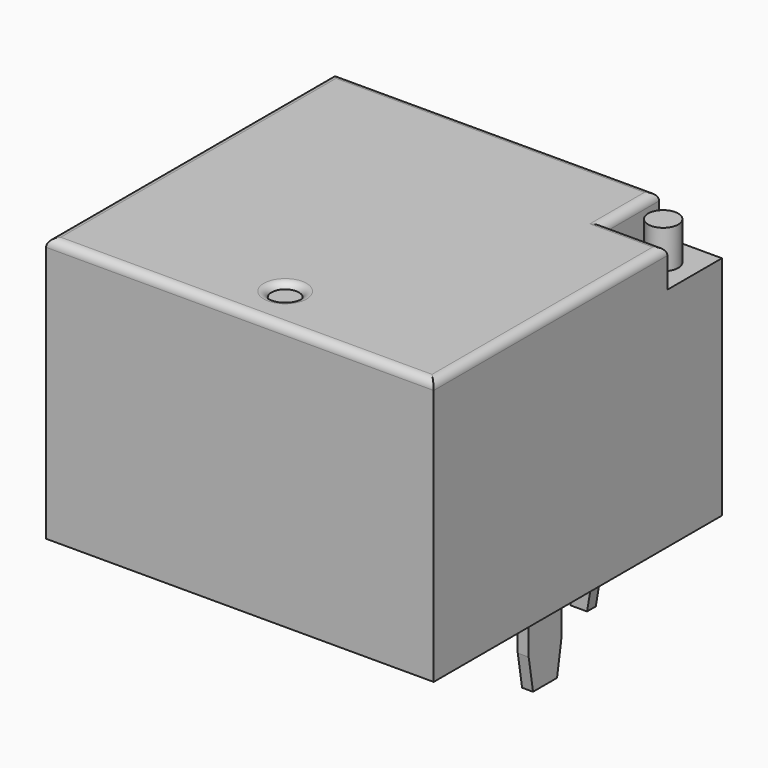
from build123d import *

# Parameters (mm, degrees)
F1_W         = 14.2
F1_H         = 13.2
F2_DEPTH     = 9.7
F0_W         = 0.4
F0_H         = 1.5
F3_DEPTH     = 3.5
F0_W_2       = 1.5
F0_H_2       = 0.4
F0_W_3       = 1
F4_W         = 2.3
F4_H         = 2.5
F4_R         = 0.55
F5_DEPTH     = 1.4
F4_R_2       = 0.5
F6_DEPTH     = 0.2
F7_T1_DEPTH  = 3.25
F7_T3_DEPTH  = 13.4
F7_T5_DEPTH  = 3.05
F7_T7_DEPTH  = 14.7
F7_T9_DEPTH  = 12.2
F7_T11_DEPTH = 15.7
F7_T19_DEPTH = 3.25
F7_T23_DEPTH = 3.05
F8_SIZE2     = 1.2
F8_SIZE      = 0.2
F8_2_SIZE2   = 1.2
F8_2_SIZE    = 0.2
F8_3_SIZE2   = 1.2
F8_3_SIZE    = 0.2
F8_4_SIZE2   = 1.2
F8_4_SIZE    = 0.2
F8_5_SIZE2   = 1.2
F8_5_SIZE    = 0.2


# Not quite as in the source:
# - a fillet or chamfer that OpenCascade refuses, or shapes differently, is made with other operations: its cross-section is extruded or revolved along the edge and cut away or added


with BuildPart() as f2:
    # F1 (on Top) → F2 (new body)
    with BuildSketch(Plane.XY):
        with Locations((-0.3, -0.5)):
            Rectangle(F1_W, F1_H)
    extrude(amount=F2_DEPTH)

    # F4 (on face) → F5 (cut)
    with BuildSketch(Plane.XY.offset(9.7)):
        with Locations((5.65, 4.85)):
            Rectangle(F4_W, F4_H)
        with Locations((5.65, 4.85)):
            Circle(F4_R, mode=Mode.SUBTRACT)
    extrude(amount=-F5_DEPTH, mode=Mode.SUBTRACT)

    # F4 (on face) → F6 (cut)
    with BuildSketch(Plane.XY.offset(9.7)):
        with Locations((0, -5.4)):
            Circle(F4_R_2)
    extrude(amount=-F6_DEPTH, mode=Mode.SUBTRACT)

    # F7: fillet of radius 0.3 on 7 edges, made by hand

    # F7_s2 → F7_t1 (cut)
    with BuildSketch(Plane.XZ.offset(-6.85)):
        with BuildLine():
            ThreePointArc((4.2, 9.7), (4.4121320344, 9.6121320344), (4.5, 9.4))
            Line((4.5, 9.4), (4.5, 9.7))
            Line((4.5, 9.7), (4.2, 9.7))
        make_face()
    extrude(amount=F7_T1_DEPTH, mode=Mode.SUBTRACT)

    # F7_s4 → F7_t3 (cut)
    with BuildSketch(Plane.YZ.offset(-8.15)):
        with BuildLine():
            ThreePointArc((6.1, 9.4), (6.0121320344, 9.6121320344), (5.8, 9.7))
            Line((5.8, 9.7), (6.1, 9.7))
            Line((6.1, 9.7), (6.1, 9.4))
        make_face()
    extrude(amount=F7_T3_DEPTH, mode=Mode.SUBTRACT)

    # F7_s6 → F7_t5 (cut)
    with BuildSketch(Plane.YZ.offset(4.5)):
        with BuildLine():
            ThreePointArc((3.3, 9.7), (3.5121320344, 9.6121320344), (3.6, 9.4))
            Line((3.6, 9.4), (3.6, 9.7))
            Line((3.6, 9.7), (3.3, 9.7))
        make_face()
    extrude(amount=F7_T5_DEPTH, mode=Mode.SUBTRACT)

    # F7_s8 → F7_t7 (cut)
    with BuildSketch(Plane.XZ.offset(-6.85)):
        with BuildLine():
            ThreePointArc((-7.4, 9.4), (-7.3121320344, 9.6121320344), (-7.1, 9.7))
            Line((-7.1, 9.7), (-7.4, 9.7))
            Line((-7.4, 9.7), (-7.4, 9.4))
        make_face()
    extrude(amount=F7_T7_DEPTH, mode=Mode.SUBTRACT)

    # F7_s10 → F7_t9 (cut)
    with BuildSketch(Plane.XZ.offset(-4.35)):
        with BuildLine():
            ThreePointArc((6.5, 9.7), (6.7121320344, 9.6121320344), (6.8, 9.4))
            Line((6.8, 9.4), (6.8, 9.7))
            Line((6.8, 9.7), (6.5, 9.7))
        make_face()
    extrude(amount=F7_T9_DEPTH, mode=Mode.SUBTRACT)

    # F7_s12 → F7_t11 (cut)
    with BuildSketch(Plane.YZ.offset(-8.15)):
        with BuildLine():
            ThreePointArc((-6.8, 9.7), (-7.0121320344, 9.6121320344), (-7.1, 9.4))
            Line((-7.1, 9.4), (-7.1, 9.7))
            Line((-7.1, 9.7), (-6.8, 9.7))
        make_face()
    extrude(amount=F7_T11_DEPTH, mode=Mode.SUBTRACT)

    # F7_s13 → F7_t14 (revolve, cut)
    with BuildSketch(Plane.XZ.offset(5.4)):
        with BuildLine():
            ThreePointArc((0.7828427125, 9.7), (0.6096376317, 9.6449489743), (0.5, 9.5))
            Line((0.5, 9.5), (0.5, 9.7))
            Line((0.5, 9.7), (0.7828427125, 9.7))
        make_face()
    revolve(axis=Axis((0, -5.4, 9.7), (0, 0, 1)), mode=Mode.SUBTRACT)


with BuildPart() as f3:
    # F0 (on Top) → F3 (new body)
    with BuildSketch(Plane.XY):
        with Locations((-5.7, 0)):
            Rectangle(F0_W, F0_H)
    extrude(amount=-F3_DEPTH)

    # F8
    f8_edges = [f3.edges().sort_by_distance(p)[0] for p in [
        (-5.7, -0.75, -3.5),
        (-5.7, 0.75, -3.5),
    ]]
    f8_side = f3.faces().sort_by_distance((-5.7, 0, -3.5))[0]
    chamfer(f8_edges, length=F8_SIZE, length2=F8_SIZE2, reference=f8_side)


with BuildPart() as f3b:
    # F0 (on Top) → F3, piece 2 (new body)
    with BuildSketch(Plane.XY):
        with Locations((5, 0)):
            Rectangle(F0_W, F0_H)
    extrude(amount=-F3_DEPTH)

    # F8#5
    f8_5_edges = [f3b.edges().sort_by_distance(p)[0] for p in [
        (5, -0.75, -3.5),
        (5, 0.75, -3.5),
    ]]
    f8_5_side = f3b.faces().sort_by_distance((5, 0, -3.5))[0]
    chamfer(f8_5_edges, length=F8_5_SIZE, length2=F8_5_SIZE2, reference=f8_5_side)


with BuildPart() as f3c:
    # F0 (on Top) → F3, piece 3 (new body)
    with BuildSketch(Plane.XY):
        with Locations((0, -5.4)):
            Rectangle(F0_W_2, F0_H_2)
    extrude(amount=-F3_DEPTH)

    # F8#2
    f8_2_edges = [f3c.edges().sort_by_distance(p)[0] for p in [
        (0.75, -5.4, -3.5),
        (-0.75, -5.4, -3.5),
    ]]
    f8_2_side = f3c.faces().sort_by_distance((0, -5.4, -3.5))[0]
    chamfer(f8_2_edges, length=F8_2_SIZE, length2=F8_2_SIZE2, reference=f8_2_side)


with BuildPart() as f3d:
    # F0 (on Top) → F3, piece 4 (new body)
    with BuildSketch(Plane.XY):
        with Locations((-3, 4.5)):
            Rectangle(F0_W_3, F0_H_2)
    extrude(amount=-F3_DEPTH)

    # F8#3
    f8_3_edges = [f3d.edges().sort_by_distance(p)[0] for p in [
        (-2.5, 4.5, -3.5),
        (-3.5, 4.5, -3.5),
    ]]
    f8_3_side = f3d.faces().sort_by_distance((-3, 4.5, -3.5))[0]
    chamfer(f8_3_edges, length=F8_3_SIZE, length2=F8_3_SIZE2, reference=f8_3_side)


with BuildPart() as f3e:
    # F0 (on Top) → F3, piece 5 (new body)
    with BuildSketch(Plane.XY):
        with Locations((3, 4.5)):
            Rectangle(F0_W_3, F0_H_2)
    extrude(amount=-F3_DEPTH)

    # F8#4
    f8_4_edges = [f3e.edges().sort_by_distance(p)[0] for p in [
        (2.5, 4.5, -3.5),
        (3.5, 4.5, -3.5),
    ]]
    f8_4_side = f3e.faces().sort_by_distance((3, 4.5, -3.5))[0]
    chamfer(f8_4_edges, length=F8_4_SIZE, length2=F8_4_SIZE2, reference=f8_4_side)


with BuildPart() as f7_tool17:
    # F7_s18 → F7_t19 (new body)
    with BuildSketch(Plane.XZ.offset(-6.1)):
        with BuildLine():
            ThreePointArc((4.2, 9.7), (4.4121320344, 9.6121320344), (4.5, 9.4))
            Line((4.5, 9.4), (4.5, 9.7))
            Line((4.5, 9.7), (4.2, 9.7))
        make_face()
    extrude(amount=F7_T19_DEPTH)

    split(bisect_by=Plane.XZ.offset(-3.6), keep=Keep.TOP)


with BuildPart() as f7_tool21:
    # F7_s22 → F7_t23 (new body)
    with BuildSketch(Plane.YZ.offset(3.75)):
        with BuildLine():
            ThreePointArc((3.3, 9.7), (3.5121320344, 9.6121320344), (3.6, 9.4))
            Line((3.6, 9.4), (3.6, 9.7))
            Line((3.6, 9.7), (3.3, 9.7))
        make_face()
    extrude(amount=F7_T23_DEPTH)

    split(bisect_by=Plane.YZ.offset(4.5), keep=Keep.BOTTOM)


with BuildPart() as f7_tool17_1:
    add(f7_tool17.part)

    # F7_t25: intersect F7_tool21
    add(f7_tool21.part, mode=Mode.INTERSECT)


with BuildPart() as f2_1:
    add(f2.part)

    # F7_t15: cut F7_tool17
    add(f7_tool17_1.part, mode=Mode.SUBTRACT)


solid = Compound([f3.part, f3b.part, f3d.part, f3e.part, f2_1.part])
